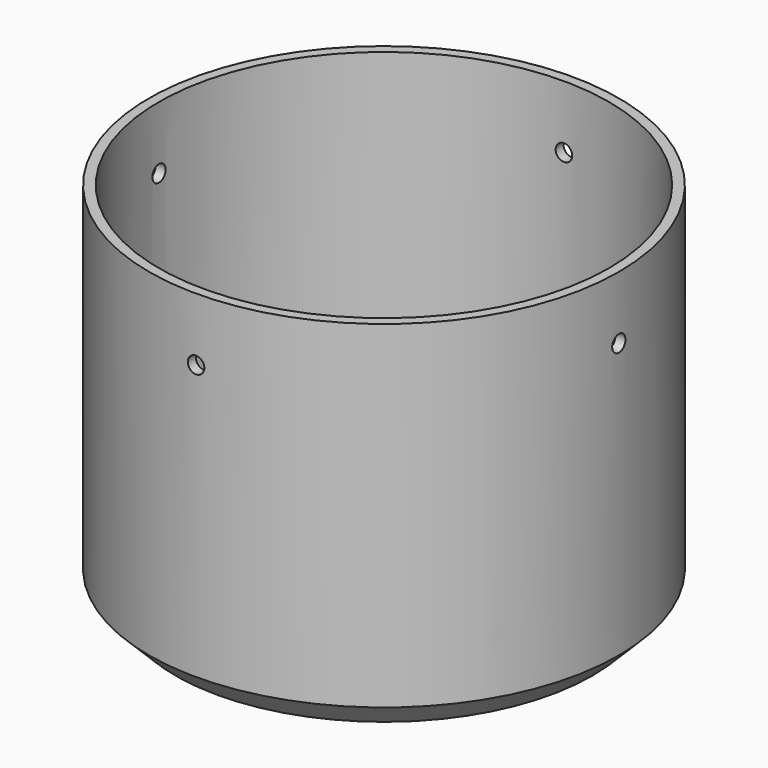
from build123d import *

# Parameters (mm, degrees)
F0_R      = 71
F1_DEPTH  = 50
F2_SIZE   = 8
F3_T      = -3
F4_R      = 2.5
F4_R_2    = 46
F5_DEPTH  = 5
F6_DEPTH  = 12.5
F9_DEPTH  = 5
F10_SIZE  = 4.99999
F11_R     = 71
F11_R_2   = 68
F12_DEPTH = 80
F13_R     = 2.5
F14_DEPTH = 75
F15_R     = 2.5
F16_DEPTH = 75


# Not quite as in the source:
# - a fillet or chamfer is up to 0.001 mm smaller than in the source, because OpenCascade refuses the exact size


with BuildPart() as f1:
    # F0 (on Top) → F1 (new body)
    with BuildSketch(Plane.XY):
        Circle(F0_R)
    extrude(amount=F1_DEPTH)

    # F2
    f2_edges = [f1.edges().sort_by_distance(p)[0] for p in [
        (-71, 0, 0),
    ]]
    chamfer(f2_edges, length=F2_SIZE)

    # F3
    f3_openings = [f1.faces().sort_by_distance(p)[0] for p in [
        (0, 0, 50),
    ]]
    offset(amount=F3_T, openings=f3_openings)

    # F4 (on face) → F5 (join)
    with BuildSketch(Plane(origin=(0, 0, 0), x_dir=(1, 0, 0), z_dir=(0, 0, -1))):
        with BuildLine():
            Line((37.5, 47.5), (-37.5, 47.5))
            ThreePointArc((-37.5, 47.5), (-40.9139438887, 46.8992014089), (-43.9176692417, 45.168997425))
            ThreePointArc((-43.9176692417, 45.168997425), (-44.5477272148, 44.5477272148), (-45.168997425, 43.9176692417))
            ThreePointArc((-45.168997425, 43.9176692417), (-46.8992014089, 40.9139438887), (-47.5, 37.5))
            Line((-47.5, 37.5), (-47.5, -37.5))
            ThreePointArc((-47.5, -37.5), (-46.8992014089, -40.9139438887), (-45.168997425, -43.9176692417))
            ThreePointArc((-45.168997425, -43.9176692417), (-44.5477272148, -44.5477272148), (-43.9176692417, -45.168997425))
            ThreePointArc((-43.9176692417, -45.168997425), (-40.9139438887, -46.8992014089), (-37.5, -47.5))
            Line((-37.5, -47.5), (37.5, -47.5))
            ThreePointArc((37.5, -47.5), (40.9139438887, -46.8992014089), (43.9176692417, -45.168997425))
            ThreePointArc((43.9176692417, -45.168997425), (44.5477272148, -44.5477272148), (45.168997425, -43.9176692417))
            ThreePointArc((45.168997425, -43.9176692417), (46.8992014089, -40.9139438887), (47.5, -37.5))
            Line((47.5, -37.5), (47.5, 37.5))
            ThreePointArc((47.5, 37.5), (46.8992014089, 40.9139438887), (45.168997425, 43.9176692417))
            ThreePointArc((45.168997425, 43.9176692417), (44.5477272148, 44.5477272148), (43.9176692417, 45.168997425))
            ThreePointArc((43.9176692417, 45.168997425), (40.9139438887, 46.8992014089), (37.5, 47.5))
        make_face()
        with Locations((-41.3657466994, -41.3657466994)):
            Circle(F4_R, mode=Mode.SUBTRACT)
        with Locations((41.3657466994, -41.3657466994)):
            Circle(F4_R, mode=Mode.SUBTRACT)
        with Locations((-41.3657466994, 41.3657466994)):
            Circle(F4_R, mode=Mode.SUBTRACT)
        Circle(F4_R_2, mode=Mode.SUBTRACT)
        with Locations((41.3657466994, 41.3657466994)):
            Circle(F4_R, mode=Mode.SUBTRACT)
        with Locations((-41.3657466994, 41.3657466994)):
            Circle(F4_R)
        with Locations((41.3657466994, 41.3657466994)):
            Circle(F4_R)
        with Locations((41.3657466994, -41.3657466994)):
            Circle(F4_R)
        with Locations((-41.3657466994, -41.3657466994)):
            Circle(F4_R)
    extrude(amount=-F5_DEPTH)

    # F4 (on face) → F6 (cut, symmetric)
    with BuildSketch(Plane(origin=(0, 0, 0), x_dir=(1, 0, 0), z_dir=(0, 0, -1))):
        with Locations((-41.3657466994, 41.3657466994)):
            Circle(F4_R)
        with Locations((41.3657466994, 41.3657466994)):
            Circle(F4_R)
        with Locations((41.3657466994, -41.3657466994)):
            Circle(F4_R)
        with Locations((-41.3657466994, -41.3657466994)):
            Circle(F4_R)
        Circle(F4_R_2)
    extrude(amount=F6_DEPTH, both=True, mode=Mode.SUBTRACT)

    # F8 (on offset) → F9 (join)
    with BuildSketch(Plane.XY.offset(25)):
        with BuildLine():
            ThreePointArc((61.4878036687, -35.5), (68.5807336665, -18.3761522023), (71, 0))
            ThreePointArc((71, 0), (50.2045814642, 50.2045814642), (0, 71))
            Line((0, 71), (0, 63))
            ThreePointArc((0, 63), (44.5477272148, 44.5477272148), (63, 0))
            ThreePointArc((63, 0), (60.8533270562, -16.3055998415), (54.5596004384, -31.5))
            Line((54.5596004384, -31.5), (61.4878036687, -35.5))
        make_face()
        with BuildLine():
            Line((0, 63), (0, 71))
            ThreePointArc((0, 71), (-61.4878036687, 35.5), (-61.4878036687, -35.5))
            Line((-61.4878036687, -35.5), (-54.5596004384, -31.5))
            ThreePointArc((-54.5596004384, -31.5), (-54.5596004384, 31.5), (0, 63))
        make_face()
        with BuildLine():
            ThreePointArc((-61.4878036687, -35.5), (0, -71), (61.4878036687, -35.5))
            Line((61.4878036687, -35.5), (54.5596004384, -31.5))
            ThreePointArc((54.5596004384, -31.5), (0, -63), (-54.5596004384, -31.5))
            Line((-54.5596004384, -31.5), (-61.4878036687, -35.5))
        make_face()
    extrude(amount=F9_DEPTH)

    # F10 (size 5 in the source; OpenCascade refuses exactly that, so slightly less here)
    f10_edges = [f1.edges().sort_by_distance(p)[0] for p in [
        (-54.5596, 31.5, 25),
    ]]
    chamfer(f10_edges, length=F10_SIZE)

    # F11 (on face) → F12 (join)
    with BuildSketch(Plane.XY.offset(30)):
        Circle(F11_R)
        Circle(F11_R_2, mode=Mode.SUBTRACT)
    extrude(amount=F12_DEPTH)

    # F13 (on Front) → F14 (cut, symmetric)
    with BuildSketch(Plane.XZ):
        with Locations((0, 91)):
            Circle(F13_R)
    extrude(amount=F14_DEPTH, both=True, mode=Mode.SUBTRACT)

    # F15 (on Right) → F16 (cut, symmetric)
    with BuildSketch(Plane.YZ):
        with Locations((0, 91)):
            Circle(F15_R)
    extrude(amount=F16_DEPTH, both=True, mode=Mode.SUBTRACT)


solid = f1.part
